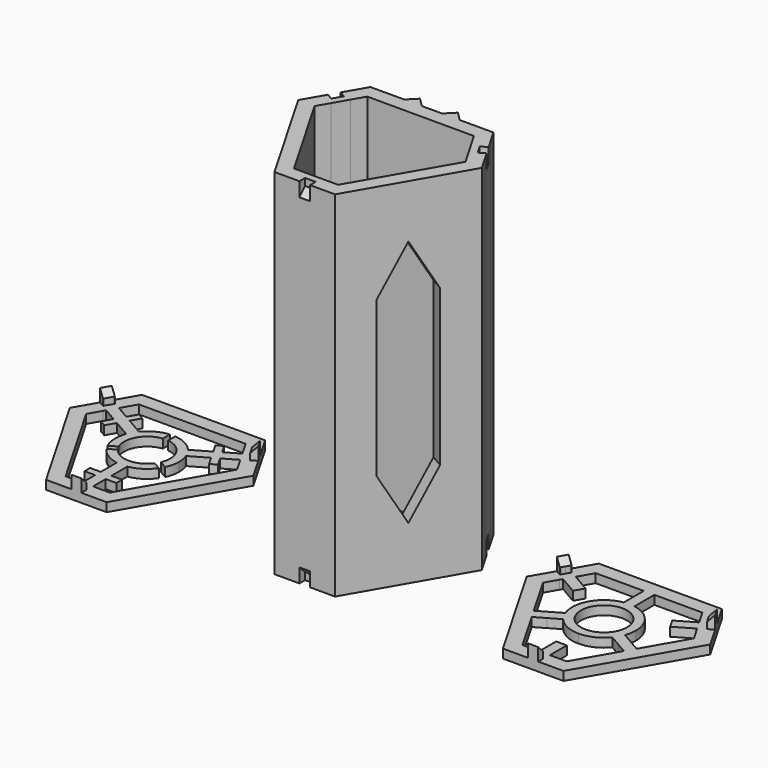
from build123d import *

# Parameters (mm, degrees)
F1_DEPTH       = 100
F0_R           = 6.5
F0_W           = 3
F0_H           = 3.4041
F0_W_2         = 1.5
F0_H_2         = 6
F2_DEPTH       = 2.5
F0_H_3         = 2
F0_H_4         = 4.5
F4_DEPTH       = 2
F3_W           = 1.5
F3_H           = 2
F5_W           = 1.5
F5_H           = 2
F6_DEPTH       = 2
F7_DEPTH       = 6.3
F8_DEPTH       = 6.3
F11_DEPTH      = 10
F12_DEPTH      = 10
F14_C1_SIZE    = 1.9999
F14_C2_SIZE    = 1.9999
F14_C3_SIZE    = 1.9999
F14_C4_SIZE    = 1.9999
F14_C5_SIZE    = 1.9999
F14_C6_SIZE    = 1.9999
F14_2_T1_DEPTH = 13.0867319519
F14_2_T3_DEPTH = 13.0867319519
F14_2_T5_DEPTH = 13.0867319519
F14_3_T1_DEPTH = 13.0867319519
F14_3_T3_DEPTH = 13.0867319519
F14_3_T5_DEPTH = 13.0867319519


# Not quite as in the source:
# - a fillet or chamfer that OpenCascade refuses, or shapes differently, is made with other operations: its cross-section is extruded or revolved along the edge and cut away or added
# - a fillet or chamfer is up to 0.001 mm smaller than in the source, because OpenCascade refuses the exact size


with BuildPart() as f1:
    # F0 (on Top) → F1 (new body)
    with BuildSketch(Plane.XY):
        Polygon((-21.6506350946, 12.5), (-23.6159910758, 9.0959035857), (-21.306589999, 5.0959035857), (-19.3412340179, 8.5), align=None)
        Polygon((-17.0318329411, 12.5), (-21.6506350946, 12.5), (-19.3412340179, 8.5), align=None)
        Polygon((-19.6852791134, 15.9040964143), (-21.6506350946, 12.5), (-17.0318329411, 12.5), (-15.0664769599, 15.9040964143), align=None)
        Polygon((-17.3758780367, 19.9040964143), (-19.6852791134, 15.9040964143), (-15.0664769599, 15.9040964143), (15.0664769599, 15.9040964143), (19.6852791134, 15.9040964143), (17.3758780367, 19.9040964143), (7.843405, 19.9040964143), (2.843405, 19.9040964143), (0, 19.9040964143), (-2.843405, 19.9040964143), (-7.843405, 19.9040964143), align=None)
        Polygon((-23.6159910758, 9.0959035857), (-25.9253921525, 5.0959035857), (-8.5495141159, -25), (-3.9307119623, -25), (-6.2401130391, -21), (-21.306589999, 5.0959035857), align=None)
        Polygon((-6.2401130391, -21), (-3.9307119623, -25), (0, -25), (-2.3094010768, -21), align=None)
        Polygon((-2.3094010768, -21), (0, -25), (2.3094010768, -21), align=None)
        Polygon((2.3094010768, -21), (0, -25), (3.9307119623, -25), (6.2401130391, -21), align=None)
        Polygon((23.6159910758, 9.0959035857), (21.6506350946, 12.5), (19.3412340179, 8.5), (21.306589999, 5.0959035857), align=None)
        Polygon((21.6506350946, 12.5), (17.0318329411, 12.5), (19.3412340179, 8.5), align=None)
        Polygon((15.0664769599, 15.9040964143), (17.0318329411, 12.5), (21.6506350946, 12.5), (19.6852791134, 15.9040964143), align=None)
        Polygon((6.2401130391, -21), (3.9307119623, -25), (8.5495141159, -25), (25.9253921525, 5.0959035857), (23.6159910758, 9.0959035857), (21.306589999, 5.0959035857), align=None)
        Polygon((-5.343405, 22.4040964143), (-7.843405, 19.9040964143), (-2.843405, 19.9040964143), align=None)
        Polygon((2.843405, 19.9040964143), (7.843405, 19.9040964143), (5.343405, 22.4040964143), align=None)
    extrude(amount=F1_DEPTH)


with BuildPart() as f2:
    # F0 (on Top) → F2 (new body)
    with BuildSketch(Plane.XY):
        Polygon((40.8986960015, 9.0959), (38.5892949248, 5.0959), (55.9651708913, -25), (60.5839730448, -25), (58.274571968, -21), (51.4913345231, -9.2510881057), (49.9913345231, -6.6530118943), (43.2080970783, 5.0959), align=None)
        Polygon((42.1640540529, 11.2875644347), (40.8986960015, 9.0959), (43.2080970783, 5.0959), (45.1734551296, 8.5), (43.9032845374, 10.7), (43.7228997797, 10.3875644347), align=None)
        Polygon((47.4828562064, 12.5), (44.9425150219, 12.5), (44.4228997797, 11.6), (46.328155668, 10.5), (47.078155668, 11.7990381057), align=None)
        Polygon((44.8294121042, 15.9041), (43.5640540529, 13.7124355653), (45.1228997797, 12.8124355653), (44.9425150219, 12.5), (47.4828562064, 12.5), (49.4482142577, 15.9041), align=None)
        Polygon((85.4653242421, 13.7124355653), (84.1999661907, 15.9041), (79.5811640372, 15.9041), (81.5465220886, 12.5), (84.086863273, 12.5), (83.9064785153, 12.8124355653), align=None)
        Polygon((84.086863273, 12.5), (81.5465220886, 12.5), (81.9512226269, 11.7990381057), (82.7012226269, 10.5), (84.6064785153, 11.6), align=None)
        Polygon((85.8212812167, 5.0959), (88.1306822934, 9.0959), (86.8653242421, 11.2875644347), (85.3064785153, 10.3875644347), (85.1260937575, 10.7), (83.8559231653, 8.5), align=None)
        Polygon((65.9146891475, -23.2), (65.9146891475, -25), (68.4454052502, -25), (70.7548063269, -21), (66.8240902242, -21), (65.553919632, -23.2), align=None)
        Polygon((70.7548063269, -21), (68.4454052502, -25), (73.0642074037, -25), (90.4400833702, 5.0959), (88.1306822934, 9.0959), (85.8212812167, 5.0959), (79.0380437718, -6.6530118943), (77.5380437718, -9.2510881057), align=None)
        Polygon((64.5146891475, -23.2), (65.553919632, -23.2), (66.8240902242, -21), (66.0146891475, -21), (64.5146891475, -21), align=None)
        Polygon((58.274571968, -21), (60.5839730448, -25), (63.1146891475, -25), (63.1146891475, -23.2), (63.4754586629, -23.2), (62.2052880707, -21), align=None)
        with BuildLine():
            ThreePointArc((56.7204605134, 4.5), (55.5462144424, 0.7526363425), (56.079476073, -3.1380217316))
            ThreePointArc((56.079476073, -3.1380217316), (56.7204605134, -4.5), (57.579476073, -5.736097943))
            ThreePointArc((57.579476073, -5.736097943), (60.6822539874, -8.1432450991), (64.5146891475, -9))
            ThreePointArc((64.5146891475, -9), (68.3471243076, -8.1432450991), (71.4499022219, -5.736097943))
            ThreePointArc((71.4499022219, -5.736097943), (72.3089177815, -4.5), (72.9499022219, -3.1380217316))
            ThreePointArc((72.9499022219, -3.1380217316), (73.372367107, -1.5942211782), (73.5146891475, 0))
            ThreePointArc((73.5146891475, 0), (73.2080215841, 2.3293714059), (72.3089177815, 4.5))
            ThreePointArc((72.3089177815, 4.5), (69.6507286925, 7.3906087566), (66.0146891475, 8.8741196746))
            ThreePointArc((66.0146891475, 8.8741196746), (64.5146891475, 9), (63.0146891475, 8.8741196746))
            ThreePointArc((63.0146891475, 8.8741196746), (59.3786496025, 7.3906087566), (56.7204605134, 4.5))
        make_face()
        with Locations((64.5146891475, 0)):
            Circle(F0_R, mode=Mode.SUBTRACT)
        with Locations((64.5146891475, 14.20205)):
            Rectangle(F0_W, F0_H)
        Polygon((47.138813181, 19.9041), (44.8294121042, 15.9041), (49.4482142577, 15.9041), (63.0146891475, 15.9041), (66.0146891475, 15.9041), (79.5811640372, 15.9041), (84.1999661907, 15.9041), (81.890565114, 19.9041), align=None)
        with BuildLine():
            Line((66.0146891475, 12.5), (63.0146891475, 12.5))
            Line((63.0146891475, 12.5), (63.0146891475, 8.8741196746))
            ThreePointArc((63.0146891475, 8.8741196746), (64.5146891475, 9), (66.0146891475, 8.8741196746))
            Line((66.0146891475, 8.8741196746), (66.0146891475, 12.5))
        make_face()
        with BuildLine():
            Line((56.079476073, -3.1380217316), (52.9393716002, -4.9509618943))
            Line((52.9393716002, -4.9509618943), (54.4393716002, -7.5490381057))
            Line((54.4393716002, -7.5490381057), (57.579476073, -5.736097943))
            ThreePointArc((57.579476073, -5.736097943), (56.7204605134, -4.5), (56.079476073, -3.1380217316))
        make_face()
        Polygon((52.9393716002, -4.9509618943), (49.9913345231, -6.6530118943), (51.4913345231, -9.2510881057), (54.4393716002, -7.5490381057), align=None)
        with BuildLine():
            Line((71.4499022219, -5.736097943), (74.5900066948, -7.5490381057))
            Line((74.5900066948, -7.5490381057), (76.0900066948, -4.9509618943))
            Line((76.0900066948, -4.9509618943), (72.9499022219, -3.1380217316))
            ThreePointArc((72.9499022219, -3.1380217316), (72.3089177815, -4.5), (71.4499022219, -5.736097943))
        make_face()
        Polygon((76.0900066948, -4.9509618943), (74.5900066948, -7.5490381057), (77.5380437718, -9.2510881057), (79.0380437718, -6.6530118943), align=None)
        Polygon((63.0146891475, -21), (62.2052880707, -21), (63.4754586629, -23.2), (64.5146891475, -23.2), (64.5146891475, -21), align=None)
        Polygon((43.9032845374, 10.7), (45.1734551296, 8.5), (45.578155668, 9.2009618943), (46.328155668, 10.5), (44.4228997797, 11.6), align=None)
        Polygon((83.4512226269, 9.2009618943), (83.8559231653, 8.5), (85.1260937575, 10.7), (84.6064785153, 11.6), (82.7012226269, 10.5), align=None)
        Polygon((83.4512226269, 9.2009618943), (82.7012226269, 10.5), (77.5050702042, 7.5), (78.2550702042, 6.2009618943), align=None)
        Polygon((82.7012226269, 10.5), (81.9512226269, 11.7990381057), (76.7550702042, 8.7990381057), (77.5050702042, 7.5), align=None)
        Polygon((47.078155668, 11.7990381057), (46.328155668, 10.5), (51.5243080907, 7.5), (52.2743080907, 8.7990381057), align=None)
        Polygon((46.328155668, 10.5), (45.578155668, 9.2009618943), (50.7743080907, 6.2009618943), (51.5243080907, 7.5), align=None)
        with Locations((63.7646891475, -18)):
            Rectangle(F0_W_2, F0_H_2)
        with Locations((65.2646891475, -18)):
            Rectangle(F0_W_2, F0_H_2)
    extrude(amount=F2_DEPTH)

    # F0 (on Top) → F8 (join)
    with BuildSketch(Plane.XY):
        Polygon((42.8640540529, 12.5), (42.1640540529, 11.2875644347), (43.7228997797, 10.3875644347), (43.9032845374, 10.7), align=None)
        Polygon((43.5640540529, 13.7124355653), (42.8640540529, 12.5), (44.9425150219, 12.5), (45.1228997797, 12.8124355653), align=None)
        Polygon((44.9425150219, 12.5), (42.8640540529, 12.5), (44.4228997797, 11.6), align=None)
        Polygon((44.4228997797, 11.6), (42.8640540529, 12.5), (43.9032845374, 10.7), align=None)
        Polygon((63.4754586629, -23.2), (64.5146891475, -25), (64.5146891475, -23.2), align=None)
        Polygon((64.5146891475, -23.2), (64.5146891475, -25), (65.553919632, -23.2), align=None)
        Polygon((65.553919632, -23.2), (64.5146891475, -25), (65.9146891475, -25), (65.9146891475, -23.2), align=None)
        Polygon((63.1146891475, -23.2), (63.1146891475, -25), (64.5146891475, -25), (63.4754586629, -23.2), align=None)
        Polygon((86.1653242421, 12.5), (85.4653242421, 13.7124355653), (83.9064785153, 12.8124355653), (84.086863273, 12.5), align=None)
        Polygon((86.1653242421, 12.5), (84.086863273, 12.5), (84.6064785153, 11.6), align=None)
        Polygon((85.1260937575, 10.7), (86.1653242421, 12.5), (84.6064785153, 11.6), align=None)
        Polygon((86.8653242421, 11.2875644347), (86.1653242421, 12.5), (85.1260937575, 10.7), (85.3064785153, 10.3875644347), align=None)
    extrude(amount=F8_DEPTH)

    # F14#3: chamfer of 2 on 3 edges, made by hand

    # F14_3_s2 → F14_3_t1 (cut)
    with BuildSketch(Plane(origin=(12.8569892989, 22.2689586981, 0), x_dir=(0, 0, 1), z_dir=(0.5, 0.8660254038, 0))):
        Polygon((6.3, 30.671359719), (4.3, 32.671359719), (6.3, 32.671359719), align=None)
    extrude(amount=F14_3_T1_DEPTH, mode=Mode.SUBTRACT)

    # F14_3_s4 → F14_3_t3 (cut)
    with BuildSketch(Plane(origin=(12.8569892989, -22.2689586981, 0), x_dir=(0, 0, 1), z_dir=(0.5, -0.8660254038, 0))):
        Polygon((6.3, -81.071359719), (4.3, -79.071359719), (6.3, -79.071359719), align=None)
    extrude(amount=F14_3_T3_DEPTH, mode=Mode.SUBTRACT)

    # F14_3_s6 → F14_3_t5 (cut)
    with BuildSketch(Plane.YZ.offset(57.9713231715)):
        Polygon((-25.2, 6.3), (-23.2, 4.3), (-23.2, 6.3), align=None)
    extrude(amount=F14_3_T5_DEPTH, mode=Mode.SUBTRACT)


with BuildPart() as f2b:
    # F0 (on Top) → F2, piece 2 (new body)
    with BuildSketch(Plane.XY):
        Polygon((-81.8725889332, 19.9040964143), (-84.1819900099, 15.9040964143), (-79.5631878564, 15.9040964143), (-49.4302339366, 15.9040964143), (-44.811431783, 15.9040964143), (-47.1208328598, 19.9040964143), align=None)
        Polygon((-84.1819900099, 15.9040964143), (-85.4473459911, 13.7124355653), (-83.8885002643, 12.8124355653), (-84.068885022, 12.5), (-81.5285438376, 12.5), (-79.5631878564, 15.9040964143), align=None)
        Polygon((-85.1081155066, 10.7), (-83.8379449143, 8.5), (-83.433244376, 9.2009618943), (-82.683244376, 10.5), (-81.933244376, 11.7990381057), (-81.5285438376, 12.5), (-84.068885022, 12.5), (-84.5885002643, 11.6), align=None)
        Polygon((-86.8473459911, 11.2875644347), (-88.1127019723, 9.0959035857), (-85.8033008955, 5.0959035857), (-83.8379449143, 8.5), (-85.1081155066, 10.7), (-85.2885002643, 10.3875644347), align=None)
        Polygon((-88.1127019723, 9.0959035857), (-90.422103049, 5.0959035857), (-73.0462250123, -25), (-68.4274228588, -25), (-70.7368239356, -21), (-85.8033008955, 5.0959035857), align=None)
        Polygon((-70.7368239356, -21), (-68.4274228588, -25), (-65.8967108965, -25), (-65.8967108965, -23.2), (-65.535941381, -23.2), (-66.8061119733, -21), align=None)
        Polygon((-65.9967108965, -21), (-66.8061119733, -21), (-65.535941381, -23.2), (-64.4967108965, -23.2), (-63.457480412, -23.2), (-62.1873098197, -21), (-62.9967108965, -21), (-64.4967108965, -21), align=None)
        Polygon((-63.0967108965, -23.2), (-63.0967108965, -25), (-60.5659989342, -25), (-58.2565978574, -21), (-62.1873098197, -21), (-63.457480412, -23.2), align=None)
        Polygon((-58.2565978574, -21), (-60.5659989342, -25), (-55.9471967806, -25), (-38.571318744, 5.0959035857), (-40.8807198207, 9.0959035857), (-43.1901208975, 5.0959035857), align=None)
        Polygon((-45.1554768786, 8.5), (-43.1901208975, 5.0959035857), (-40.8807198207, 9.0959035857), (-42.1460758019, 11.2875644347), (-43.7049215287, 10.3875644347), (-43.8853062864, 10.7), align=None)
        Polygon((-44.924536771, 12.5), (-47.4648779554, 12.5), (-47.060177417, 11.7990381057), (-46.310177417, 10.5), (-45.560177417, 9.2009618943), (-45.1554768786, 8.5), (-43.8853062864, 10.7), (-44.4049215287, 11.6), align=None)
        with BuildLine():
            ThreePointArc((-57.561497822, 5.736097943), (-60.3280124385, 7.976337077), (-63.7467108965, 8.9686955573))
            Line((-63.7467108965, 8.9686955573), (-63.7467108965, 6.4565857851))
            ThreePointArc((-63.7467108965, 6.4565857851), (-59.6425889368, 4.3229041164), (-57.9967108965, 0))
            ThreePointArc((-57.9967108965, 0), (-58.1314659081, -1.3166838031), (-58.5301435849, -2.5787738397))
            Line((-58.5301435849, -2.5787738397), (-56.354592705, -3.8348287258))
            ThreePointArc((-56.354592705, -3.8348287258), (-55.713799542, -1.9648074049), (-55.4967108965, 0))
            ThreePointArc((-55.4967108965, 0), (-55.6390329369, 1.5942211782), (-56.061497822, 3.1380217316))
            ThreePointArc((-56.061497822, 3.1380217316), (-56.7024822624, 4.5), (-57.561497822, 5.736097943))
        make_face()
        with BuildLine():
            ThreePointArc((-72.931923971, 3.1380217316), (-73.4887706633, -0.3779697731), (-72.6388290879, -3.8348287258))
            Line((-72.6388290879, -3.8348287258), (-70.4632782081, -2.5787738397))
            ThreePointArc((-70.4632782081, -2.5787738397), (-70.1258760211, 3.25), (-65.2467108965, 6.4565857851))
            Line((-65.2467108965, 6.4565857851), (-65.2467108965, 8.9686955573))
            ThreePointArc((-65.2467108965, 8.9686955573), (-68.6654093545, 7.976337077), (-71.431923971, 5.736097943))
            ThreePointArc((-71.431923971, 5.736097943), (-72.2909395306, 4.5), (-72.931923971, 3.1380217316))
        make_face()
        with BuildLine():
            Line((-69.7132782081, -3.8778119454), (-71.8888290879, -5.1338668315))
            ThreePointArc((-71.8888290879, -5.1338668315), (-69.3200722053, -7.5983673039), (-65.9967108965, -8.8741196746))
            ThreePointArc((-65.9967108965, -8.8741196746), (-64.4967108965, -9), (-62.9967108965, -8.8741196746))
            ThreePointArc((-62.9967108965, -8.8741196746), (-59.6733495877, -7.5983673039), (-57.104592705, -5.1338668315))
            Line((-57.104592705, -5.1338668315), (-59.2801435849, -3.8778119454))
            ThreePointArc((-59.2801435849, -3.8778119454), (-64.4967108965, -6.5), (-69.7132782081, -3.8778119454))
        make_face()
        with BuildLine():
            Line((-78.7861300589, 8.25), (-79.5361300589, 6.9509618943))
            Line((-79.5361300589, 6.9509618943), (-77.8040792514, 5.9509618943))
            Line((-77.8040792514, 5.9509618943), (-72.931923971, 3.1380217316))
            ThreePointArc((-72.931923971, 3.1380217316), (-72.2909395306, 4.5), (-71.431923971, 5.736097943))
            Line((-71.431923971, 5.736097943), (-76.3040792514, 8.5490381057))
            Line((-76.3040792514, 8.5490381057), (-78.0361300589, 9.5490381057))
            Line((-78.0361300589, 9.5490381057), (-78.7861300589, 8.25))
        make_face()
        with BuildLine():
            Line((-52.6893425416, 8.5490381057), (-57.561497822, 5.736097943))
            ThreePointArc((-57.561497822, 5.736097943), (-56.7024822624, 4.5), (-56.061497822, 3.1380217316))
            Line((-56.061497822, 3.1380217316), (-51.1893425416, 5.9509618943))
            Line((-51.1893425416, 5.9509618943), (-49.457291734, 6.9509618943))
            Line((-49.457291734, 6.9509618943), (-50.207291734, 8.25))
            Line((-50.207291734, 8.25), (-50.957291734, 9.5490381057))
            Line((-50.957291734, 9.5490381057), (-52.6893425416, 8.5490381057))
        make_face()
        with BuildLine():
            Line((-65.9967108965, -14.5), (-65.9967108965, -16.5))
            Line((-65.9967108965, -16.5), (-64.4967108965, -16.5))
            Line((-64.4967108965, -16.5), (-62.9967108965, -16.5))
            Line((-62.9967108965, -16.5), (-62.9967108965, -14.5))
            Line((-62.9967108965, -14.5), (-62.9967108965, -8.8741196746))
            ThreePointArc((-62.9967108965, -8.8741196746), (-64.4967108965, -9), (-65.9967108965, -8.8741196746))
            Line((-65.9967108965, -8.8741196746), (-65.9967108965, -14.5))
        make_face()
        Polygon((-81.933244376, 11.7990381057), (-82.683244376, 10.5), (-78.7861300589, 8.25), (-78.0361300589, 9.5490381057), align=None)
        Polygon((-82.683244376, 10.5), (-83.433244376, 9.2009618943), (-79.5361300589, 6.9509618943), (-78.7861300589, 8.25), align=None)
        Polygon((-77.8040792514, 5.9509618943), (-79.5361300589, 6.9509618943), (-81.0361300589, 4.352885683), (-79.3040792514, 3.352885683), align=None)
        Polygon((-76.5361300589, 12.147114317), (-78.0361300589, 9.5490381057), (-76.3040792514, 8.5490381057), (-74.8040792514, 11.147114317), align=None)
        Polygon((-52.6893425416, 8.5490381057), (-50.957291734, 9.5490381057), (-52.457291734, 12.147114317), (-54.1893425416, 11.147114317), align=None)
        Polygon((-49.457291734, 6.9509618943), (-51.1893425416, 5.9509618943), (-49.6893425416, 3.352885683), (-47.957291734, 4.352885683), align=None)
        with Locations((-61.4967108965, -15.5)):
            Rectangle(F0_W, F0_H_3)
        with Locations((-67.4967108965, -15.5)):
            Rectangle(F0_W, F0_H_3)
        with Locations((-65.2467108965, -18.75)):
            Rectangle(F0_W_2, F0_H_4)
        with Locations((-63.7467108965, -18.75)):
            Rectangle(F0_W_2, F0_H_4)
        Polygon((-46.310177417, 10.5), (-47.060177417, 11.7990381057), (-50.957291734, 9.5490381057), (-50.207291734, 8.25), align=None)
        Polygon((-45.560177417, 9.2009618943), (-46.310177417, 10.5), (-50.207291734, 8.25), (-49.457291734, 6.9509618943), align=None)
        Polygon((-44.811431783, 15.9040964143), (-49.4302339366, 15.9040964143), (-47.4648779554, 12.5), (-44.924536771, 12.5), (-45.1049215287, 12.8124355653), (-43.5460758019, 13.7124355653), align=None)
    extrude(amount=F2_DEPTH)

    # F0 (on Top) → F7 (join)
    with BuildSketch(Plane.XY):
        Polygon((-86.1473459911, 12.5), (-86.8473459911, 11.2875644347), (-85.2885002643, 10.3875644347), (-85.1081155066, 10.7), align=None)
        Polygon((-84.5885002643, 11.6), (-86.1473459911, 12.5), (-85.1081155066, 10.7), align=None)
        Polygon((-84.068885022, 12.5), (-86.1473459911, 12.5), (-84.5885002643, 11.6), align=None)
        Polygon((-85.4473459911, 13.7124355653), (-86.1473459911, 12.5), (-84.068885022, 12.5), (-83.8885002643, 12.8124355653), align=None)
        Polygon((-65.8967108965, -23.2), (-65.8967108965, -25), (-64.4967108965, -25), (-65.535941381, -23.2), align=None)
        Polygon((-64.4967108965, -23.2), (-64.4967108965, -25), (-63.457480412, -23.2), align=None)
        Polygon((-65.535941381, -23.2), (-64.4967108965, -25), (-64.4967108965, -23.2), align=None)
        Polygon((-63.457480412, -23.2), (-64.4967108965, -25), (-63.0967108965, -25), (-63.0967108965, -23.2), align=None)
        Polygon((-42.8460758019, 12.5), (-44.924536771, 12.5), (-44.4049215287, 11.6), align=None)
        Polygon((-43.8853062864, 10.7), (-42.8460758019, 12.5), (-44.4049215287, 11.6), align=None)
        Polygon((-42.1460758019, 11.2875644347), (-42.8460758019, 12.5), (-43.8853062864, 10.7), (-43.7049215287, 10.3875644347), align=None)
        Polygon((-42.8460758019, 12.5), (-43.5460758019, 13.7124355653), (-45.1049215287, 12.8124355653), (-44.924536771, 12.5), align=None)
    extrude(amount=F7_DEPTH)

    # F14#2: chamfer of 2 on 3 edges, made by hand

    # F14_2_s2 → F14_2_t1 (cut)
    with BuildSketch(Plane(origin=(-19.3958607121, -33.5946162099, 0), x_dir=(0, 0, 1), z_dir=(0.5, 0.8660254038, 0))):
        Polygon((4.3, -79.0557900969), (6.3, -81.0557900969), (6.3, -79.0557900969), align=None)
    extrude(amount=F14_2_T1_DEPTH, mode=Mode.SUBTRACT)

    # F14_2_s4 → F14_2_t3 (cut)
    with BuildSketch(Plane.YZ.offset(-71.0400768724)):
        Polygon((-23.2, 4.3), (-25.2, 6.3), (-23.2, 6.3), align=None)
    extrude(amount=F14_2_T3_DEPTH, mode=Mode.SUBTRACT)

    # F14_2_s6 → F14_2_t5 (cut)
    with BuildSketch(Plane(origin=(-19.3958607121, 33.5946162099, 0), x_dir=(0, 0, 1), z_dir=(0.5, -0.8660254038, 0))):
        Polygon((4.3, 32.6557900969), (6.3, 30.6557900969), (6.3, 32.6557900969), align=None)
    extrude(amount=F14_2_T5_DEPTH, mode=Mode.SUBTRACT)


with BuildPart() as f4:
    # F3 (on face) → F4 (new body)
    with BuildSketch(Plane.XY.offset(100)):
        Polygon((-20.9006350946, 13.7990381057), (-21.6506350946, 12.5), (-19.918584287, 11.5), (-19.168584287, 12.7990381057), align=None)
        Polygon((-21.6506350946, 12.5), (-22.4006350946, 11.2009618943), (-20.668584287, 10.2009618943), (-19.918584287, 11.5), align=None)
    extrude(amount=-F4_DEPTH)


with BuildPart() as f4b:
    # F3 (on face) → F4, piece 2 (new body)
    with BuildSketch(Plane.XY.offset(100)):
        Polygon((19.918584287, 11.5), (21.6506350946, 12.5), (20.9006350946, 13.7990381057), (19.168584287, 12.7990381057), align=None)
        Polygon((20.668584287, 10.2009618943), (22.4006350946, 11.2009618943), (21.6506350946, 12.5), (19.918584287, 11.5), align=None)
    extrude(amount=-F4_DEPTH)


with BuildPart() as f4c:
    # F3 (on face) → F4, piece 3 (new body)
    with BuildSketch(Plane.XY.offset(100)):
        with Locations((0.75, -24)):
            Rectangle(F3_W, F3_H)
        with Locations((-0.75, -24)):
            Rectangle(F3_W, F3_H)
    extrude(amount=-F4_DEPTH)


with BuildPart() as f6:
    # F5 (on face) → F6 (new body)
    with BuildSketch(Plane(origin=(0, 0, 0), x_dir=(1, 0, 0), z_dir=(0, 0, -1))):
        with Locations((-0.75, 24)):
            Rectangle(F5_W, F5_H)
        with Locations((0.75, 24)):
            Rectangle(F5_W, F5_H)
    extrude(amount=-F6_DEPTH)


with BuildPart() as f6b:
    # F5 (on face) → F6, piece 2 (new body)
    with BuildSketch(Plane(origin=(0, 0, 0), x_dir=(1, 0, 0), z_dir=(0, 0, -1))):
        Polygon((21.6506350946, -12.5), (22.4006350946, -11.2009618943), (20.668584287, -10.2009618943), (19.918584287, -11.5), align=None)
        Polygon((20.9006350946, -13.7990381057), (21.6506350946, -12.5), (19.918584287, -11.5), (19.168584287, -12.7990381057), align=None)
    extrude(amount=-F6_DEPTH)


with BuildPart() as f6c:
    # F5 (on face) → F6, piece 3 (new body)
    with BuildSketch(Plane(origin=(0, 0, 0), x_dir=(1, 0, 0), z_dir=(0, 0, -1))):
        Polygon((-20.668584287, -10.2009618943), (-22.4006350946, -11.2009618943), (-21.6506350946, -12.5), (-19.918584287, -11.5), align=None)
        Polygon((-19.918584287, -11.5), (-21.6506350946, -12.5), (-20.9006350946, -13.7990381057), (-19.168584287, -12.7990381057), align=None)
    extrude(amount=-F6_DEPTH)


with BuildPart() as f11:
    # F9 (on face) → F11 (new body)
    with BuildSketch(Plane(origin=(-17.2374531342, -9.9520482072, 0), x_dir=(0.5, -0.8660254038, 0), z_dir=(-0.8660254038, -0.5, 0))):
        Polygon((0, 85), (-7.5, 72.0096189432), (-7.5, 27.9903810568), (0, 15), (7.5, 27.9903810568), (7.5, 72.0096189432), align=None)
    extrude(amount=-F11_DEPTH)


with BuildPart() as f12:
    # F10 (on face) → F12 (new body)
    with BuildSketch(Plane(origin=(17.2374531342, -9.9520482072, 0), x_dir=(0.5, 0.8660254038, 0), z_dir=(0.8660254038, -0.5, 0))):
        Polygon((0, 85), (-7.5, 72.0096189432), (-7.5, 27.9903810568), (0, 15), (7.5, 27.9903810568), (7.5, 72.0096189432), align=None)
    extrude(amount=-F12_DEPTH)


with BuildPart() as f1_1:
    add(f1.part)

    # F13: cut F4, F4b, F4c, F6, F6c, F6b, F11, F12
    add(f4.part, mode=Mode.SUBTRACT)
    add(f4b.part, mode=Mode.SUBTRACT)
    add(f4c.part, mode=Mode.SUBTRACT)
    add(f6.part, mode=Mode.SUBTRACT)
    add(f6c.part, mode=Mode.SUBTRACT)
    add(f6b.part, mode=Mode.SUBTRACT)
    add(f11.part, mode=Mode.SUBTRACT)
    add(f12.part, mode=Mode.SUBTRACT)

    # F14: chamfer of 2 on 6 edges, made by hand

    # F14_c1 (size 2 in the source; OpenCascade refuses exactly that, so slightly less here)
    f14_c1_edges = [f1_1.edges().sort_by_distance(p)[0] for p in [
        (21.6506350946, 12.5, 2),
    ]]
    chamfer(f14_c1_edges, length=F14_C1_SIZE)

    # F14_c2 (size 2 in the source; OpenCascade refuses exactly that, so slightly less here)
    f14_c2_edges = [f1_1.edges().sort_by_distance(p)[0] for p in [
        (21.6506350946, 12.5, 98),
    ]]
    chamfer(f14_c2_edges, length=F14_C2_SIZE)

    # F14_c3 (size 2 in the source; OpenCascade refuses exactly that, so slightly less here)
    f14_c3_edges = [f1_1.edges().sort_by_distance(p)[0] for p in [
        (0, -25, 2),
    ]]
    chamfer(f14_c3_edges, length=F14_C3_SIZE)

    # F14_c4 (size 2 in the source; OpenCascade refuses exactly that, so slightly less here)
    f14_c4_edges = [f1_1.edges().sort_by_distance(p)[0] for p in [
        (0, -25, 98),
    ]]
    chamfer(f14_c4_edges, length=F14_C4_SIZE)

    # F14_c5 (size 2 in the source; OpenCascade refuses exactly that, so slightly less here)
    f14_c5_edges = [f1_1.edges().sort_by_distance(p)[0] for p in [
        (-21.6506350946, 12.5, 2),
    ]]
    chamfer(f14_c5_edges, length=F14_C5_SIZE)

    # F14_c6 (size 2 in the source; OpenCascade refuses exactly that, so slightly less here)
    f14_c6_edges = [f1_1.edges().sort_by_distance(p)[0] for p in [
        (-21.6506350946, 12.5, 98),
    ]]
    chamfer(f14_c6_edges, length=F14_C6_SIZE)


solid = Compound([f2.part, f2b.part, f1_1.part])
